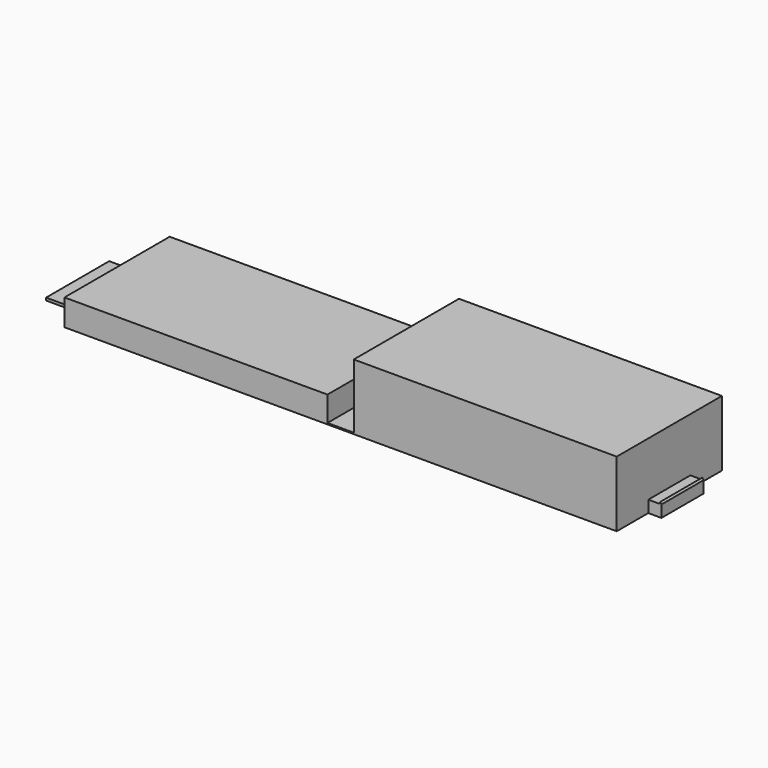
from build123d import *

# Parameters (mm, degrees)
F0_W        = 100
F0_H        = 50
F1_DEPTH    = 25
F2_W        = 10
F2_H        = 50
F3_DEPTH    = 0.5
F4_W        = 100
F4_H        = 50
F5_DEPTH    = 10
F6_T        = 2.5
F6_T3_DEPTH = 55
F7_R        = 5
F8_W        = 5
F8_H        = 20
F9_DEPTH    = 4.5
F10_W       = 15
F10_H       = 30
F10_W_2     = 5
F10_H_2     = 20
F11_DEPTH   = 1
F13_DEPTH   = 10


# Not quite as in the source:
# - a shell that OpenCascade refuses in one call is made with other operations: the cavity is built on its own and cut out


with BuildPart() as f1:
    # F0 (on Top) → F1 (new body)
    with BuildSketch(Plane.XY):
        Rectangle(F0_W, F0_H)
    extrude(amount=F1_DEPTH)

    # F2 (on Top) → F3 (join)
    with BuildSketch(Plane.XY):
        with Locations((-55, 0)):
            Rectangle(F2_W, F2_H)
    extrude(amount=F3_DEPTH)

    # F4 (on Top) → F5 (join)
    with BuildSketch(Plane.XY):
        with Locations((-110, 0)):
            Rectangle(F4_W, F4_H)
    extrude(amount=F5_DEPTH)

    # F6: shell of thickness 2.5, made by hand


with BuildPart() as f6_core1:
    # F6_t2: copy of F1
    add(f1.part)

    # the walls: a layer under each face that stays
    f6_faces = [f6_core1.faces().sort_by_distance(p)[0] for p in [
        (-50, 0, 12.75),
        (15, 25, 20.8333333333),
        (-160, 0, 5),
        (-110, 0, 10),
        (-60, 0, 5.25),
        (50, 0, 12.5),
        (0, 0, 25),
        (-125, -25, 4.1666666667),
        (-55, 0, 0.5),
    ]]
    thicken(f6_faces, amount=-F6_T, mode=Mode.SUBTRACT)

    # F6_s4 → F6_t3 (cut)
    with BuildSketch(Plane.XZ.offset(-27.5)):
        Polygon((-50.025, 0.525), (-47.5, 0.5), (-47.5, -2), (-50, -2), align=None)
        Polygon((-59.975, 0.525), (-62.5, 0.5), (-62.5, -2), (-60, -2), align=None)
    extrude(amount=F6_T3_DEPTH, mode=Mode.SUBTRACT)


with BuildPart() as f1_1:
    add(f1.part)

    # what is left inside the walls is the cavity
    f6_cavity = [f6_core1.part.solids().sort_by_distance(p)[0] for p in [
        (0, -7.5, 22.475),
        (-110, -7.5, 7.475),
    ]]
    add(f6_cavity, mode=Mode.SUBTRACT)

    # F7
    f7_edges = [f1_1.edges().sort_by_distance(p)[0] for p in [
        (-157.5, -22.5, 3.75),
        (-62.5, -22.5, 3.75),
        (-62.5, 22.5, 3.75),
        (-157.5, 22.5, 3.75),
        (-47.5, -22.5, 11.25),
        (47.5, -22.5, 11.25),
        (47.5, 22.5, 11.25),
        (-47.5, 22.5, 11.25),
    ]]
    fillet(f7_edges, radius=F7_R)

    # F8 (on Top) → F9 (join)
    with BuildSketch(Plane.XY):
        with Locations((52.5, 0)):
            Rectangle(F8_W, F8_H)
    extrude(amount=F9_DEPTH)

    # F10 (on Top) → F11 (join)
    with BuildSketch(Plane.XY):
        with Locations((-167.5, 0)):
            Rectangle(F10_W, F10_H)
        with Locations((-167.5, 0)):
            Rectangle(F10_W_2, F10_H_2, mode=Mode.SUBTRACT)
    extrude(amount=F11_DEPTH)

    # F12 (on Front) → F13 (join, symmetric)
    with BuildSketch(Plane.XZ):
        Polygon((55, 4.5), (54.5669872981, 5.25), (54.1339745962, 4.5), align=None)
    extrude(amount=F13_DEPTH, both=True)


solid = f1_1.part
